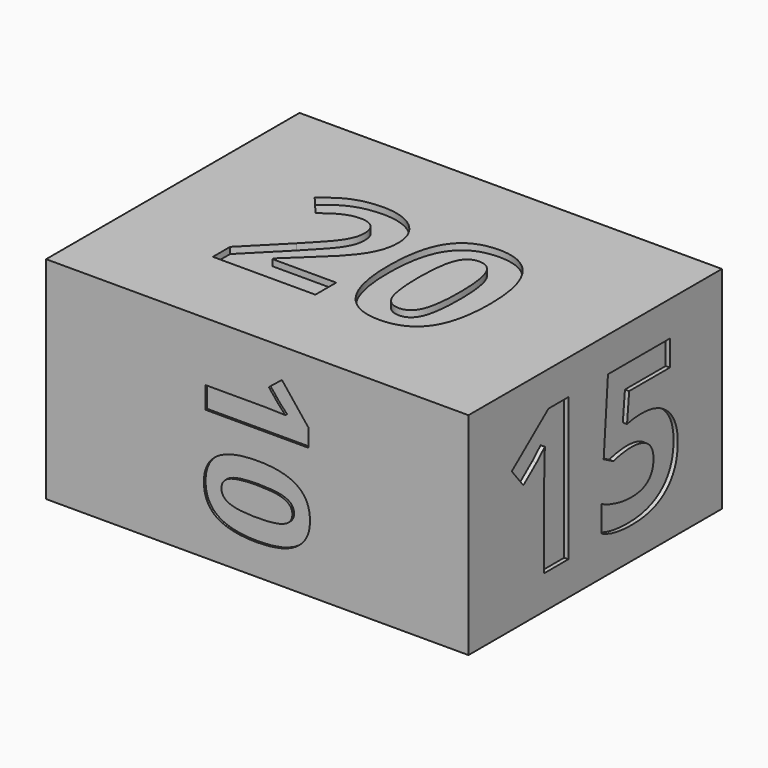
from build123d import *

# Parameters (mm, degrees)
F0_W         = 20
F0_H         = 15
F1_DEPTH     = 5
F2_TEXT_SIZE = 9.4700026903
F3_DEPTH     = 0.2
F4_TEXT_SIZE = 6.8330441746
F5_DEPTH     = 0.1
F6_TEXT_SIZE = 9.7222222222
F7_DEPTH     = 0.3


# Not quite as in the source:
# - Text() gives the source's letters only with a copy of the font that has no kerning and outlines rounded to 1/6400 em; it was checked with that copy


with BuildPart() as f1:
    # F0 (on Top) → F1 (new body, symmetric)
    with BuildSketch(Plane.XY):
        Rectangle(F0_W, F0_H)
    extrude(amount=F1_DEPTH, both=True)

    # F2 (on face) → F3 (cut)
    with BuildSketch(Plane.YZ.offset(10)):
        with Locations((-5.5, -3.4092009685)):
            Text('15', F2_TEXT_SIZE, font='Open Sans', font_style=FontStyle.BOLD, text_align=(TextAlign.LEFT, TextAlign.BOTTOM))
    extrude(amount=-F3_DEPTH, mode=Mode.SUBTRACT)

    # F4 (on face) → F5 (cut)
    with BuildSketch(Plane.XZ.offset(7.5)):
        with Locations(Location((-2.4598959028, 4), (0, 0, -90))):
            Text('10', F4_TEXT_SIZE, font='Open Sans', font_style=FontStyle.BOLD, text_align=(TextAlign.LEFT, TextAlign.BOTTOM))
    extrude(amount=-F5_DEPTH, mode=Mode.SUBTRACT)

    # F6 (on face) → F7 (cut)
    with BuildSketch(Plane.XY.offset(5)):
        with Locations((-5.6912977431, -3.5)):
            Text('20', F6_TEXT_SIZE, font='Open Sans', font_style=FontStyle.BOLD, text_align=(TextAlign.LEFT, TextAlign.BOTTOM))
    extrude(amount=-F7_DEPTH, mode=Mode.SUBTRACT)


solid = f1.part
